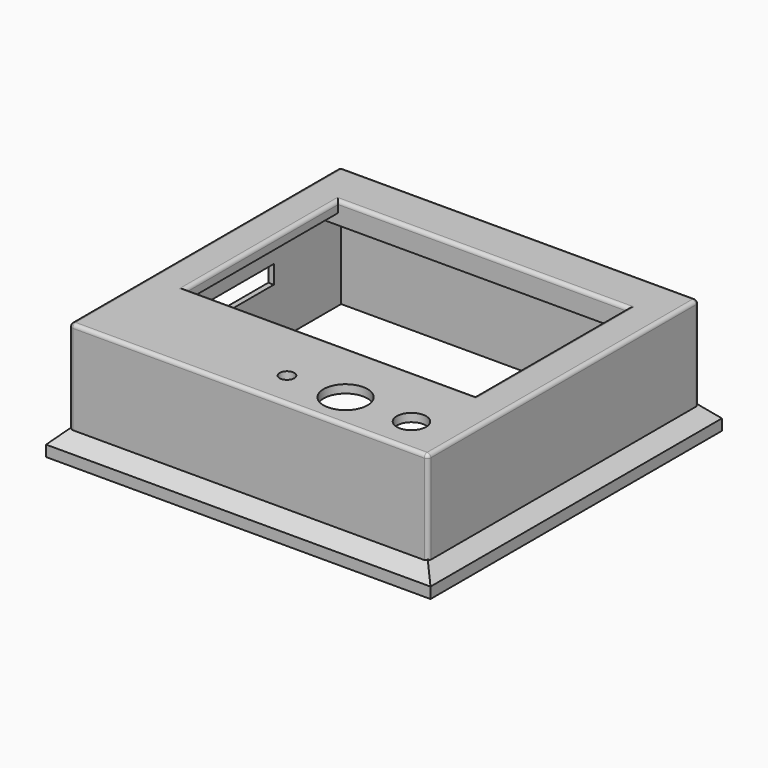
from build123d import *

# Parameters (mm, degrees)
F1_DEPTH  = 6
F0_W      = 8
F0_H      = 52
F2_DEPTH  = 3
F0_W_2    = 98
F0_H_2    = 92.5
F3_DEPTH  = 32
F5_W      = 28
F5_H      = 5
F6_DEPTH  = 20
F0_W_3    = 95
F0_H_3    = 23.5
F0_R      = 2
F0_R_2    = 6
F0_R_3    = 4
F7_DEPTH  = 2.25
F9_W      = 105
F9_H      = 99.5
F9_W_2    = 95
F9_H_2    = 89.5
F10_DEPTH = 3
F11_SIZE  = 3.49999
F12_R     = 1


# Not quite as in the source:
# - a fillet or chamfer is up to 0.001 mm smaller than in the source, because OpenCascade refuses the exact size
# - a feature names something its author has since deleted; it is built from what else it names


with BuildPart() as f1:
    # F0 (on Top) → F1 (new body)
    with BuildSketch(Plane.XY):
        Polygon((0, 52), (0, 0), (-79, 0), (-87, 0), (-87, -3), (8, -3), (8, 63), (-87, 63), (-87, 52), (-79, 52), align=None)
    extrude(amount=-F1_DEPTH)

    # F0 (on Top) → F2 (join)
    with BuildSketch(Plane.XY):
        with Locations((-83, 26)):
            Rectangle(F0_W, F0_H)
    extrude(amount=-F2_DEPTH)

    # F0 (on Top) → F3 (join)
    with BuildSketch(Plane.XY):
        with Locations((-39.5, 18.25)):
            Rectangle(F0_W_2, F0_H_2)
        Polygon((-87, -3), (-87, 0), (-87, 52), (-87, 63), (8, 63), (8, -3), (8, -26.5), (-87, -26.5), align=None, mode=Mode.SUBTRACT)
    extrude(amount=-F3_DEPTH)

    # F5 (on offset) → F6 (cut)
    with BuildSketch(Plane.YZ.offset(-88.5)):
        with Locations((26, -15.5)):
            Rectangle(F5_W, F5_H)
    extrude(amount=F6_DEPTH, mode=Mode.SUBTRACT)

    # F0 (on Top) → F7 (join)
    with BuildSketch(Plane.XY):
        with Locations((-39.5, -14.75)):
            Rectangle(F0_W_3, F0_H_3)
        with Locations((-37, -18)):
            Circle(F0_R, mode=Mode.SUBTRACT)
        with Locations((-21, -18)):
            Circle(F0_R_2, mode=Mode.SUBTRACT)
        with Locations((-3, -18)):
            Circle(F0_R_3, mode=Mode.SUBTRACT)
    extrude(amount=-F7_DEPTH)

    # F9 (on offset) → F10 (join)
    with BuildSketch(Plane.XY.offset(-32)):
        with Locations((-39.5, 18.25)):
            Rectangle(F9_W, F9_H)
        with Locations((-39.5, 18.25)):
            Rectangle(F9_W_2, F9_H_2, mode=Mode.SUBTRACT)
    extrude(amount=F10_DEPTH)

    # F11 (size 3.5 in the source; OpenCascade refuses exactly that, so slightly less here)
    f11_edges = [f1.edges().sort_by_distance(p)[0] for p in [
        (-88.5, 18.25, -29),
        (-39.5, -28, -29),
        (9.5, 18.25, -29),
        (-39.5, 64.5, -29),
    ]]
    chamfer(f11_edges, length=F11_SIZE)

    # F12
    f12_edges = [f1.edges().sort_by_distance(p)[0] for p in [
        (-88.5, -28, -12.750005),
        (-39.5, -28, 0),
        (-88.5, 18.25, 0),
        (-39.5, 64.5, 0),
        (9.5, 18.25, 0),
        (0, 26, 0),
        (-39.5, 0, 0),
        (-79, 26, 0),
        (-39.5, 52, 0),
        (9.5, -28, -12.750005),
        (9.5, 64.5, -12.750005),
        (-88.5, 64.5, -12.750005),
    ]]
    fillet(f12_edges, radius=F12_R)


solid = f1.part
